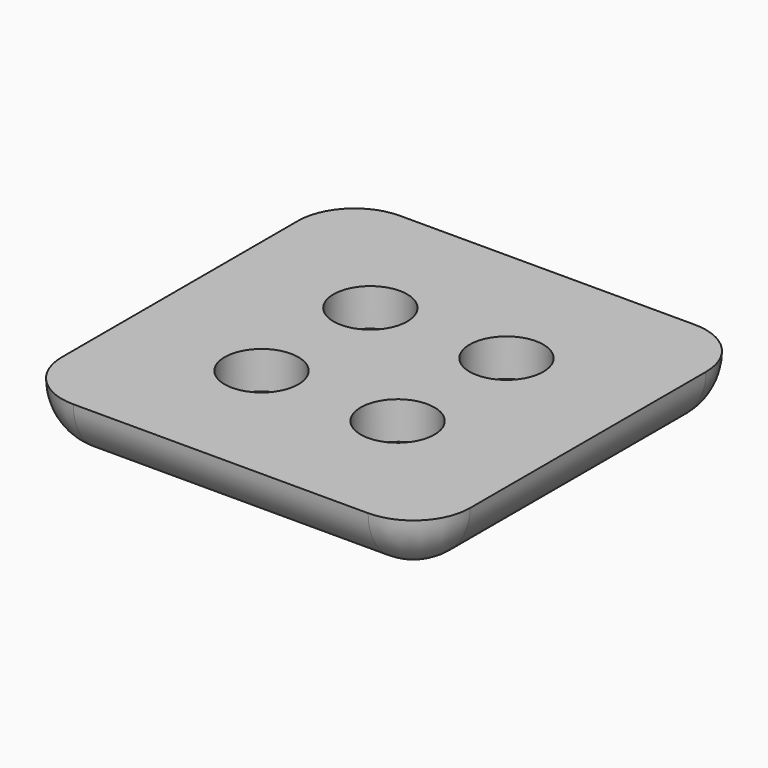
from build123d import *

# Parameters (mm, degrees)
F0_W     = 36
F0_H     = 36
F1_DEPTH = 2.5
F2_R     = 3.25
F3_DEPTH = 3.3
F4_R     = 5
F5_R     = 4.99999


# Not quite as in the source:
# - a fillet or chamfer is up to 0.001 mm smaller than in the source, because OpenCascade refuses the exact size


with BuildPart() as f1:
    # F0 (on Top) → F1 (new body, symmetric)
    with BuildSketch(Plane.XY):
        Rectangle(F0_W, F0_H)
    extrude(amount=F1_DEPTH, both=True)

    # F2 (on face) → F3 (cut)
    with BuildSketch(Plane.XY.offset(2.5)):
        with Locations((-6, 6)):
            Circle(F2_R)
        with Locations((6, 6)):
            Circle(F2_R)
        with Locations((6, -6)):
            Circle(F2_R)
        with Locations((-6, -6)):
            Circle(F2_R)
    extrude(amount=-F3_DEPTH, mode=Mode.SUBTRACT)

    # F4
    f4_edges = [f1.edges().sort_by_distance(p)[0] for p in [
        (-18, -18, 0),
        (-18, 18, 0),
        (18, -18, 0),
        (18, 18, 0),
    ]]
    fillet(f4_edges, radius=F4_R)

    # F5 (radius 5 in the source; OpenCascade refuses exactly that, so slightly less here)
    f5_edges = [f1.edges().sort_by_distance(p)[0] for p in [
        (0, 18, -2.5),
    ]]
    fillet(f5_edges, radius=F5_R)


solid = f1.part
